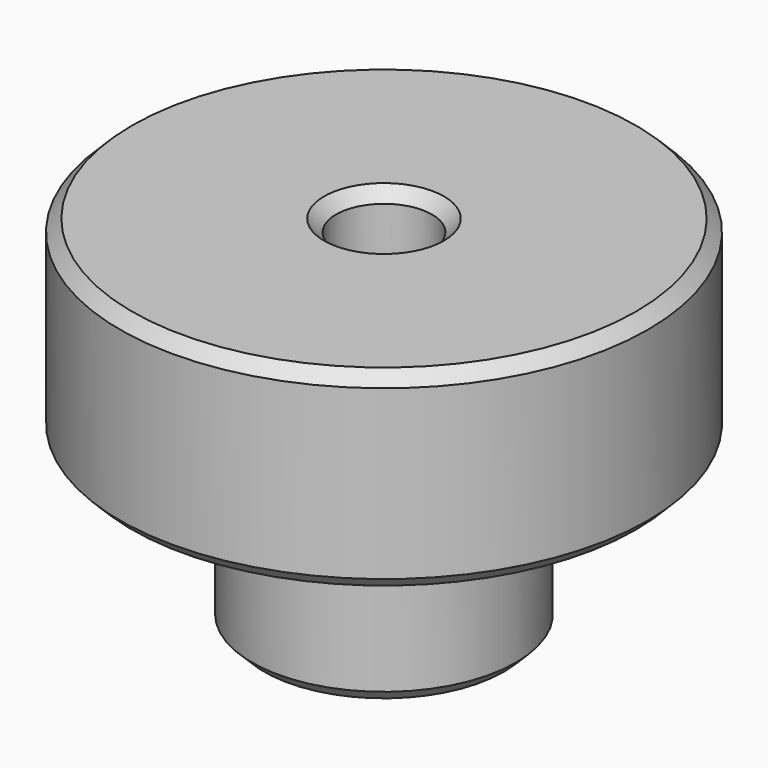
from build123d import *

# Parameters (mm, degrees)
F2_R     = 2
F3_DEPTH = 10.001
F4_SIZE  = 0.5
F5_R     = 2
F6_DEPTH = 25
F7_SIZE  = 0.5
F8_R     = 0.99999


# Not quite as in the source:
# - a fillet or chamfer is up to 0.001 mm smaller than in the source, because OpenCascade refuses the exact size


with BuildPart() as f1:
    # F0 (on Front) → F1 (revolve)
    with BuildSketch(Plane.XZ):
        with BuildLine():
            Line((3.5, 10.4850548723), (0, 10.4850548723))
            Line((0, 10.4850548723), (0, 0.4850548723))
            Line((0, 0.4850548723), (5.5, 0.4850548723))
            Line((5.5, 0.4850548723), (5.5, 8.4850548723))
            ThreePointArc((5.5, 8.4850548723), (4.9142135624, 9.8992684347), (3.5, 10.4850548723))
        make_face()
    revolve(axis=Axis((0, 0, 5.4850548723), (0, 0, -1)))

    # F2 (on face) → F3 (cut, through all)
    with BuildSketch(Plane.XY.offset(10.4850548723)):
        Circle(F2_R)
    extrude(amount=-F3_DEPTH, mode=Mode.SUBTRACT)

    # F4
    f4_edges = [f1.edges().sort_by_distance(p)[0] for p in [
        (-5.5, 0, 0.485055),
        (-2, 0, 0.485055),
    ]]
    chamfer(f4_edges, length=F4_SIZE)


with BuildPart() as f1b:
    # F0 (on Front) → F1, piece 2 (revolve)
    with BuildSketch(Plane.XZ):
        with BuildLine():
            Line((0, 11.4850548723), (3.5, 11.4850548723))
            ThreePointArc((3.5, 11.4850548723), (5.6213203436, 10.6063752159), (6.5, 8.4850548723))
            Line((6.5, 8.4850548723), (6.5, 7.4850548723))
            Line((6.5, 7.4850548723), (11, 7.4850548723))
            Line((11, 7.4850548723), (11, 15.4850548723))
            Line((11, 15.4850548723), (0, 15.4850548723))
            Line((0, 15.4850548723), (0, 11.4850548723))
        make_face()
    revolve(axis=Axis((0, 0, 5.4850548723), (0, 0, -1)))

    # F5 (on face) → F6 (cut)
    with BuildSketch(Plane.XY.offset(15.4850548723)):
        Circle(F5_R)
    extrude(amount=-F6_DEPTH, mode=Mode.SUBTRACT)

    # F7
    f7_edges = [f1b.edges().sort_by_distance(p)[0] for p in [
        (-11, 0, 7.485055),
        (-11, 0, 15.485055),
        (-2, 0, 15.485055),
    ]]
    chamfer(f7_edges, length=F7_SIZE)

    # F8 (radius 1 in the source; OpenCascade refuses exactly that, so slightly less here)
    f8_edges = [f1b.edges().sort_by_distance(p)[0] for p in [
        (-6.5, 0, 7.485055),
    ]]
    fillet(f8_edges, radius=F8_R)


solid = Compound([f1.part, f1b.part])
